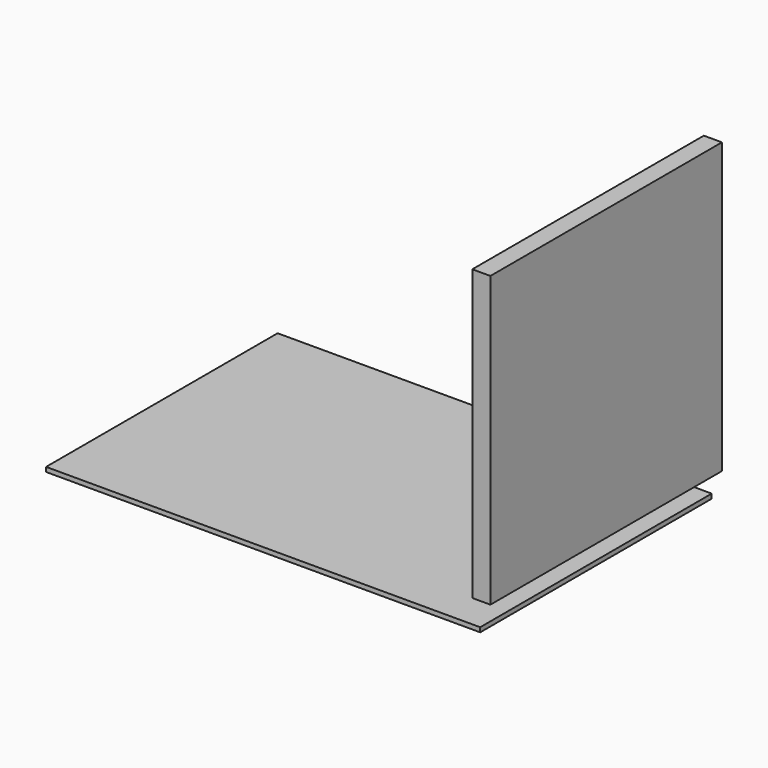
from build123d import *

# Parameters (mm, degrees)
F0_W     = 304.8
F0_H     = 203.2
F1_DEPTH = 3.175
F2_W     = 12.7
F2_H     = 203.2
F3_DEPTH = 101.6


# Not quite as in the source:
# - a feature names something its author has since deleted; it is built from what else it names


with BuildPart() as f1:
    # F0 (on Top) → F1 (new body)
    with BuildSketch(Plane.XY):
        Rectangle(F0_W, F0_H)
    extrude(amount=F1_DEPTH)


with BuildPart() as f3:
    # F2 (on Front) → F3 (new body, symmetric)
    with BuildSketch(Plane.XZ):
        with Locations((153.2097309828, 121.0248197005)):
            Rectangle(F2_W, F2_H)
    extrude(amount=F3_DEPTH, both=True)


solid = Compound([f1.part, f3.part])
